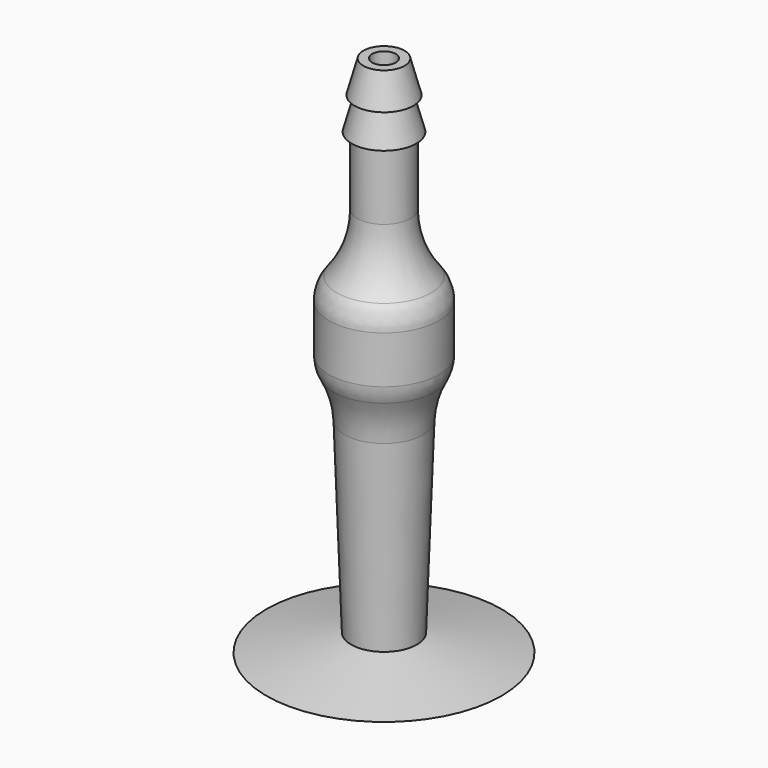
from build123d import *

# Parameters (mm, degrees)
F3_R = 3


# Not quite as in the source:
# - a fillet or chamfer that OpenCascade refuses, or shapes differently, is made with other operations: its cross-section is extruded or revolved along the edge and cut away or added


with BuildPart() as f1:
    # F0 (on Front) → F1 (revolve)
    with BuildSketch(Plane.XZ):
        Polygon((-1, 0), (-1, 20), (-1.75, 20), (-2.5, 17.25), (-2, 17.25), (-2.75, 14.5), (-2.25, 14.5), (-2.25, 3), (-4.6620704234, 3), (-4.6620704234, -3), (-3.5, -3), (-2.8, -23), (-1.6, -23), align=None)
        Polygon((0, -23), (-1.6, -23), (-2.8, -23), (-10, -24.5), (0, -24.5), align=None)
    revolve(axis=Axis((0, 0, 10), (0, 0, 1)))

    # F2: fillet of radius 8 on 2 edges, made by hand

    # F2_s1 → F2_t2 (revolve)
    with BuildSketch(Plane.XZ):
        with BuildLine():
            ThreePointArc((-2.25, 8.7249491741), (-2.8776382138, 5.6187808443), (-4.6620704234, 3))
            Line((-4.6620704234, 3), (-4.5503118318, 2.8855010165))
            ThreePointArc((-4.5503118318, 2.8855010165), (-3.4560352117, 2.84), (-2.25, 2.84))
            Line((-2.25, 2.84), (-2.09, 3))
            Line((-2.09, 3), (-2.09, 8.7249491741))
            Line((-2.09, 8.7249491741), (-2.25, 8.7249491741))
        make_face()
    revolve(axis=Axis((0, 0, 3), (0, 0, 1)))

    # F2_s3 → F2_t4 (revolve)
    with BuildSketch(Plane.XZ):
        with BuildLine():
            ThreePointArc((-4.6620704234, -3), (-3.7272345044, -4.9644393238), (-3.3562164627, -7.1081010661))
            Line((-3.3562164627, -7.1081010661), (-3.1963143727, -7.102504493))
            Line((-3.1963143727, -7.102504493), (-3.3400979101, -2.9944034269))
            Line((-3.3400979101, -2.9944034269), (-3.5, -2.84))
            ThreePointArc((-3.5, -2.84), (-4.0810352117, -2.84), (-4.5282854126, -2.9122414055))
            Line((-4.5282854126, -2.9122414055), (-4.6620704234, -3))
        make_face()
    revolve(axis=Axis((0, 0, -3), (0, 0, 1)))

    # F3
    f3_edges = [f1.edges().sort_by_distance(p)[0] for p in [
        (4.66207, 0, 3),
        (4.66207, 0, -3),
    ]]
    fillet(f3_edges, radius=F3_R)


solid = f1.part
